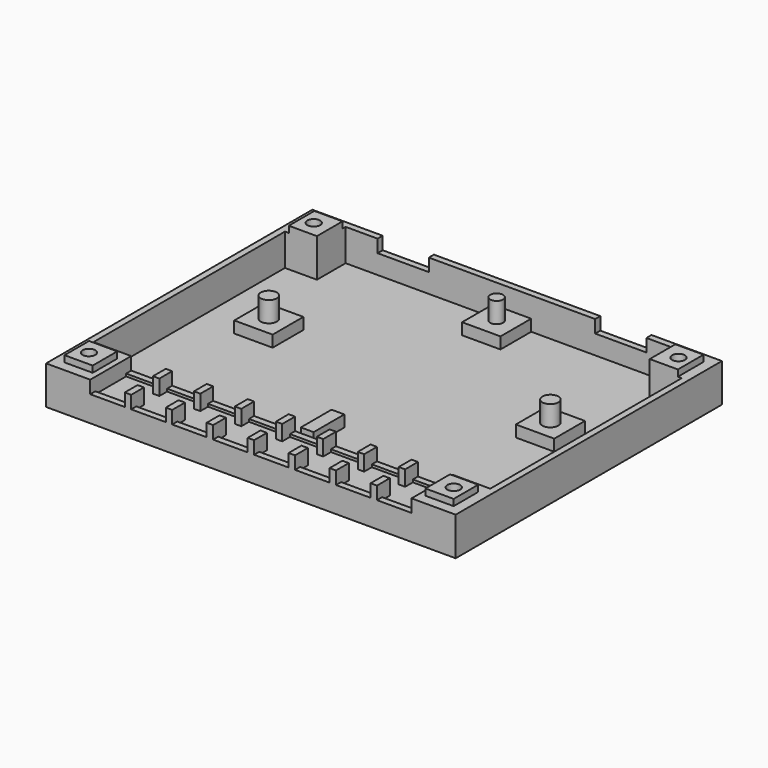
from build123d import *

# Parameters (mm, degrees)
F0_W          = 6.858
F0_H          = 3.81
F0_H_2        = 1.905
F0_W_2        = 1.27
F0_W_3        = 10.16
F0_H_3        = 13.335
F0_W_4        = 7.62
F0_H_4        = 7.62
F0_R          = 1.5875
F0_W_5        = 5.588
F0_H_5        = 6.096
F0_H_6        = 1.27
F0_R_2        = 1.27
F0_W_6        = 0.762
F0_H_7        = 6.35
F0_W_7        = 2.54
F1_DEPTH      = 5.08
F2_DEPTH      = 3.81
F3_DEPTH      = 1.524
F4_DEPTH      = 2.54
F5_DEPTH      = 2.54
F6_DEPTH      = 0.508
F7_DEPTH      = 3.81
F8_DEPTH      = 3.81
F8_DEPTH_BACK = 3.81


# Not quite as in the source:
# - a feature names something its author has since deleted; it is built from what else it names


with BuildPart() as f1:
    # F0 (on Top) → F1 (new body)
    with BuildSketch(Plane.XY):
        with Locations((4.064, -34.29)):
            Rectangle(F0_W, F0_H)
        with Locations((-20.32, -31.4325)):
            Rectangle(F0_W, F0_H_2)
        with Locations((28.448, -34.29)):
            Rectangle(F0_W, F0_H)
        with Locations((4.064, -37.1475)):
            Rectangle(F0_W, F0_H_2)
        with Locations((-4.064, -37.1475)):
            Rectangle(F0_W, F0_H_2)
        with Locations((0, -34.29)):
            Rectangle(F0_W_2, F0_H)
        with Locations((4.064, -31.4325)):
            Rectangle(F0_W, F0_H_2)
        with Locations((-4.064, -34.29)):
            Rectangle(F0_W, F0_H)
        with Locations((21.59, 18.7325)):
            Rectangle(F0_W_3, F0_H_3)
        with Locations((-21.59, 18.7325)):
            Rectangle(F0_W_3, F0_H_3)
        with Locations((-27.94, 0)):
            Rectangle(F0_W_4, F0_H_4)
        with Locations((-27.94, 0)):
            Circle(F0_R, mode=Mode.SUBTRACT)
        with Locations((27.94, 0)):
            Rectangle(F0_W_4, F0_H_4)
        with Locations((27.94, 0)):
            Circle(F0_R, mode=Mode.SUBTRACT)
        with Locations((-12.192, -37.1475)):
            Rectangle(F0_W, F0_H_2)
        Polygon((-3.81, 25.4), (-6.35, 25.4), (-16.51, 25.4), (-16.51, 12.065), (-26.67, 12.065), (-26.67, 25.4), (-31.75, 25.4), (-31.75, 3.81), (-24.13, 3.81), (-24.13, -3.81), (-31.75, -3.81), (-31.75, -25.4), (-1.27, -25.4), (-1.27, -17.78), (1.27, -17.78), (1.27, -25.4), (31.75, -25.4), (31.75, -3.81), (24.13, -3.81), (24.13, 3.81), (31.75, 3.81), (31.75, 25.4), (26.67, 25.4), (26.67, 12.065), (16.51, 12.065), (16.51, 25.4), (6.35, 25.4), (3.81, 25.4), (3.81, 17.78), (-3.81, 17.78), align=None)
        with Locations((-4.064, -31.4325)):
            Rectangle(F0_W, F0_H_2)
        with Locations((-16.256, -37.1475)):
            Rectangle(F0_W_2, F0_H_2)
        with Locations((-12.192, -34.29)):
            Rectangle(F0_W, F0_H)
        Polygon((40.64, 26.67), (26.67, 26.67), (26.67, 25.4), (31.75, 25.4), (33.02, 25.4), (39.37, 25.4), (39.37, 24.638), (39.37, 18.288), (39.37, -29.21), (31.877, -29.21), (31.877, -30.48), (39.37, -30.48), (39.37, -38.1), (31.877, -38.1), (31.877, -39.37), (40.64, -39.37), align=None)
        with Locations((-20.32, -37.1475)):
            Rectangle(F0_W, F0_H_2)
        with Locations((-20.32, -34.29)):
            Rectangle(F0_W, F0_H)
        Polygon((31.877, -36.195), (31.877, -38.1), (39.37, -38.1), (39.37, -30.48), (31.877, -30.48), (31.877, -32.385), align=None)
        with Locations((35.814, -34.29)):
            Rectangle(F0_W_5, F0_H_5, mode=Mode.SUBTRACT)
        with Locations((-12.192, -31.4325)):
            Rectangle(F0_W, F0_H_2)
        with Locations((12.192, -38.735)):
            Rectangle(F0_W, F0_H_6)
        with Locations((28.448, -38.735)):
            Rectangle(F0_W, F0_H_6)
        with Locations((28.448, -31.4325)):
            Rectangle(F0_W, F0_H_2)
        with Locations((-24.384, -34.29)):
            Rectangle(F0_W_2, F0_H)
        with Locations((20.32, -38.735)):
            Rectangle(F0_W, F0_H_6)
        with Locations((0, 21.59)):
            Rectangle(F0_W_4, F0_H_4)
        with Locations((0, 21.59)):
            Circle(F0_R_2, mode=Mode.SUBTRACT)
        with Locations((28.448, -37.1475)):
            Rectangle(F0_W, F0_H_2)
        with Locations((12.192, -37.1475)):
            Rectangle(F0_W, F0_H_2)
        with Locations((16.256, -34.29)):
            Rectangle(F0_W_2, F0_H)
        with Locations((-12.192, -38.735)):
            Rectangle(F0_W, F0_H_6)
        with Locations((-28.448, -31.4325)):
            Rectangle(F0_W, F0_H_2)
        with Locations((4.064, -38.735)):
            Rectangle(F0_W, F0_H_6)
        with Locations((20.32, -31.4325)):
            Rectangle(F0_W, F0_H_2)
        with Locations((20.32, -37.1475)):
            Rectangle(F0_W, F0_H_2)
        with Locations((12.192, -34.29)):
            Rectangle(F0_W, F0_H)
        with Locations((-20.32, -38.735)):
            Rectangle(F0_W, F0_H_6)
        with Locations((-28.448, -29.845)):
            Rectangle(F0_W, F0_H_6)
        with Locations((12.192, -31.4325)):
            Rectangle(F0_W, F0_H_2)
        with Locations((20.32, -34.29)):
            Rectangle(F0_W, F0_H)
        with Locations((-4.064, -38.735)):
            Rectangle(F0_W, F0_H_6)
        with Locations((12.192, -29.845)):
            Rectangle(F0_W, F0_H_6)
        with Locations((8.128, -34.29)):
            Rectangle(F0_W_2, F0_H)
        with Locations((0, -37.1475)):
            Rectangle(F0_W_2, F0_H_2)
        with Locations((24.384, -31.4325)):
            Rectangle(F0_W_2, F0_H_2)
        with Locations((4.064, -29.845)):
            Rectangle(F0_W, F0_H_6)
        with Locations((-38.989, 21.463)):
            Rectangle(F0_W_6, F0_H_7)
        with Locations((-35.814, 21.463)):
            Rectangle(F0_W_5, F0_H_7)
        with Locations((-36.195, 21.463)):
            Circle(F0_R_2, mode=Mode.SUBTRACT)
        with Locations((0, -21.59)):
            Rectangle(F0_W_7, F0_H_4)
        with Locations((38.989, 21.463)):
            Rectangle(F0_W_6, F0_H_7)
        with Locations((35.814, 21.463)):
            Rectangle(F0_W_5, F0_H_7)
        with Locations((36.195, 21.463)):
            Circle(F0_R_2, mode=Mode.SUBTRACT)
        with Locations((0, -31.4325)):
            Rectangle(F0_W_2, F0_H_2)
        with Locations((-8.128, -34.29)):
            Rectangle(F0_W_2, F0_H)
        with Locations((16.256, -37.1475)):
            Rectangle(F0_W_2, F0_H_2)
        with Locations((-4.064, -29.845)):
            Rectangle(F0_W, F0_H_6)
        with Locations((-16.256, -34.29)):
            Rectangle(F0_W_2, F0_H)
        with Locations((21.59, 26.035)):
            Rectangle(F0_W_3, F0_H_6)
        with Locations((-24.384, -37.1475)):
            Rectangle(F0_W_2, F0_H_2)
        with Locations((-21.59, 26.035)):
            Rectangle(F0_W_3, F0_H_6)
        with Locations((11.43, 26.035)):
            Rectangle(F0_W_3, F0_H_6)
        with Locations((-12.192, -29.845)):
            Rectangle(F0_W, F0_H_6)
        with Locations((-11.43, 26.035)):
            Rectangle(F0_W_3, F0_H_6)
        Polygon((-6.35, 26.67), (-6.35, 25.4), (-3.81, 25.4), (3.81, 25.4), (6.35, 25.4), (6.35, 26.67), align=None)
        with Locations((28.448, -29.845)):
            Rectangle(F0_W, F0_H_6)
        with Locations((16.256, -31.4325)):
            Rectangle(F0_W_2, F0_H_2)
        with Locations((24.384, -34.29)):
            Rectangle(F0_W_2, F0_H)
        with Locations((-20.32, -29.845)):
            Rectangle(F0_W, F0_H_6)
        with Locations((-24.384, -31.4325)):
            Rectangle(F0_W_2, F0_H_2)
        with Locations((20.32, -29.845)):
            Rectangle(F0_W, F0_H_6)
        with Locations((24.384, -37.1475)):
            Rectangle(F0_W_2, F0_H_2)
        with Locations((24.384, -29.845)):
            Rectangle(F0_W_2, F0_H_6)
        with Locations((24.384, -38.735)):
            Rectangle(F0_W_2, F0_H_6)
        with Locations((16.256, -29.845)):
            Rectangle(F0_W_2, F0_H_6)
        with Locations((16.256, -38.735)):
            Rectangle(F0_W_2, F0_H_6)
        with Locations((8.128, -29.845)):
            Rectangle(F0_W_2, F0_H_6)
        with Locations((-8.128, -37.1475)):
            Rectangle(F0_W_2, F0_H_2)
        with Locations((0, -29.845)):
            Rectangle(F0_W_2, F0_H_6)
        with Locations((8.128, -38.735)):
            Rectangle(F0_W_2, F0_H_6)
        with Locations((0, 21.59)):
            Circle(F0_R_2)
        with Locations((27.94, 0)):
            Circle(F0_R)
        with Locations((-27.94, 0)):
            Circle(F0_R)
        with Locations((0, -38.735)):
            Rectangle(F0_W_2, F0_H_6)
        with Locations((-8.128, -29.845)):
            Rectangle(F0_W_2, F0_H_6)
        with Locations((-16.256, -29.845)):
            Rectangle(F0_W_2, F0_H_6)
        with Locations((-8.128, -38.735)):
            Rectangle(F0_W_2, F0_H_6)
        with Locations((-16.256, -38.735)):
            Rectangle(F0_W_2, F0_H_6)
        with Locations((8.128, -31.4325)):
            Rectangle(F0_W_2, F0_H_2)
        with Locations((-8.128, -31.4325)):
            Rectangle(F0_W_2, F0_H_2)
        with Locations((-24.384, -38.735)):
            Rectangle(F0_W_2, F0_H_6)
        with Locations((-16.256, -31.4325)):
            Rectangle(F0_W_2, F0_H_2)
        with Locations((8.128, -37.1475)):
            Rectangle(F0_W_2, F0_H_2)
        with Locations((-24.384, -29.845)):
            Rectangle(F0_W_2, F0_H_6)
        with Locations((-28.448, -38.735)):
            Rectangle(F0_W, F0_H_6)
        Polygon((-31.75, 3.81), (-31.75, 25.4), (-33.02, 25.4), (-33.02, 24.638), (-33.02, 18.288), (-38.608, 18.288), (-39.37, 18.288), (-39.37, -29.21), (-31.877, -29.21), (-25.019, -29.21), (-23.749, -29.21), (-16.891, -29.21), (-15.621, -29.21), (-8.763, -29.21), (-7.493, -29.21), (-0.635, -29.21), (0.635, -29.21), (7.493, -29.21), (8.763, -29.21), (15.621, -29.21), (16.891, -29.21), (23.749, -29.21), (25.019, -29.21), (31.877, -29.21), (39.37, -29.21), (39.37, 18.288), (38.608, 18.288), (33.02, 18.288), (33.02, 24.638), (33.02, 25.4), (31.75, 25.4), (31.75, 3.81), (31.75, -3.81), (31.75, -25.4), (1.27, -25.4), (-1.27, -25.4), (-31.75, -25.4), (-31.75, -3.81), align=None)
        Polygon((-31.75, 25.4), (-26.67, 25.4), (-26.67, 26.67), (-40.64, 26.67), (-40.64, -39.37), (-31.877, -39.37), (-31.877, -38.1), (-39.37, -38.1), (-39.37, -30.48), (-31.877, -30.48), (-31.877, -29.21), (-39.37, -29.21), (-39.37, 18.288), (-39.37, 24.638), (-39.37, 25.4), (-33.02, 25.4), align=None)
        with Locations((-28.448, -37.1475)):
            Rectangle(F0_W, F0_H_2)
        with Locations((-28.448, -34.29)):
            Rectangle(F0_W, F0_H)
        Polygon((-39.37, -38.1), (-31.877, -38.1), (-31.877, -36.195), (-31.877, -32.385), (-31.877, -30.48), (-39.37, -30.48), align=None)
        with Locations((-35.814, -34.29)):
            Rectangle(F0_W_5, F0_H_5, mode=Mode.SUBTRACT)
        with Locations((-35.814, -34.29)):
            Rectangle(F0_W_5, F0_H_5)
        with Locations((-36.195, -34.29)):
            Circle(F0_R_2, mode=Mode.SUBTRACT)
        with Locations((35.814, -34.29)):
            Rectangle(F0_W_5, F0_H_5)
        with Locations((36.195, -34.29)):
            Circle(F0_R_2, mode=Mode.SUBTRACT)
        with Locations((-36.195, -34.29)):
            Circle(F0_R_2)
        with Locations((36.195, -34.29)):
            Circle(F0_R_2)
        Polygon((-33.02, 24.638), (-33.02, 25.4), (-39.37, 25.4), (-39.37, 24.638), (-38.608, 24.638), align=None)
        Polygon((39.37, 25.4), (33.02, 25.4), (33.02, 24.638), (38.608, 24.638), (39.37, 24.638), align=None)
        with Locations((-36.195, 21.463)):
            Circle(F0_R_2)
        with Locations((36.195, 21.463)):
            Circle(F0_R_2)
    extrude(amount=-F1_DEPTH)

    # F0 (on Top) → F2 (cut)
    with BuildSketch(Plane.XY):
        Polygon((-3.81, 25.4), (-6.35, 25.4), (-16.51, 25.4), (-16.51, 12.065), (-26.67, 12.065), (-26.67, 25.4), (-31.75, 25.4), (-31.75, 3.81), (-24.13, 3.81), (-24.13, -3.81), (-31.75, -3.81), (-31.75, -25.4), (-1.27, -25.4), (-1.27, -17.78), (1.27, -17.78), (1.27, -25.4), (31.75, -25.4), (31.75, -3.81), (24.13, -3.81), (24.13, 3.81), (31.75, 3.81), (31.75, 25.4), (26.67, 25.4), (26.67, 12.065), (16.51, 12.065), (16.51, 25.4), (6.35, 25.4), (3.81, 25.4), (3.81, 17.78), (-3.81, 17.78), align=None)
        with Locations((-21.59, 18.7325)):
            Rectangle(F0_W_3, F0_H_3)
        with Locations((21.59, 18.7325)):
            Rectangle(F0_W_3, F0_H_3)
        Polygon((-31.75, 3.81), (-31.75, 25.4), (-33.02, 25.4), (-33.02, 24.638), (-33.02, 18.288), (-38.608, 18.288), (-39.37, 18.288), (-39.37, -29.21), (-31.877, -29.21), (-25.019, -29.21), (-23.749, -29.21), (-16.891, -29.21), (-15.621, -29.21), (-8.763, -29.21), (-7.493, -29.21), (-0.635, -29.21), (0.635, -29.21), (7.493, -29.21), (8.763, -29.21), (15.621, -29.21), (16.891, -29.21), (23.749, -29.21), (25.019, -29.21), (31.877, -29.21), (39.37, -29.21), (39.37, 18.288), (38.608, 18.288), (33.02, 18.288), (33.02, 24.638), (33.02, 25.4), (31.75, 25.4), (31.75, 3.81), (31.75, -3.81), (31.75, -25.4), (1.27, -25.4), (-1.27, -25.4), (-31.75, -25.4), (-31.75, -3.81), align=None)
    extrude(amount=-F2_DEPTH, mode=Mode.SUBTRACT)

    # F0 (on Top) → F3 (cut)
    with BuildSketch(Plane.XY):
        with Locations((-27.94, 0)):
            Rectangle(F0_W_4, F0_H_4)
        with Locations((-27.94, 0)):
            Circle(F0_R, mode=Mode.SUBTRACT)
        with Locations((0, 21.59)):
            Rectangle(F0_W_4, F0_H_4)
        with Locations((0, 21.59)):
            Circle(F0_R_2, mode=Mode.SUBTRACT)
        with Locations((27.94, 0)):
            Rectangle(F0_W_4, F0_H_4)
        with Locations((27.94, 0)):
            Circle(F0_R, mode=Mode.SUBTRACT)
        with Locations((0, -21.59)):
            Rectangle(F0_W_7, F0_H_4)
    extrude(amount=-F3_DEPTH, mode=Mode.SUBTRACT)

    # F0 (on Top) → F4 (join)
    with BuildSketch(Plane.XY):
        with Locations((-27.94, 0)):
            Circle(F0_R)
        with Locations((27.94, 0)):
            Circle(F0_R)
        with Locations((0, 21.59)):
            Circle(F0_R_2)
        with Locations((-11.43, 26.035)):
            Rectangle(F0_W_3, F0_H_6)
        Polygon((-6.35, 26.67), (-6.35, 25.4), (-3.81, 25.4), (3.81, 25.4), (6.35, 25.4), (6.35, 26.67), align=None)
        with Locations((11.43, 26.035)):
            Rectangle(F0_W_3, F0_H_6)
    extrude(amount=F4_DEPTH)

    # F0 (on Top) → F5 (join)
    with BuildSketch(Plane.XY):
        Polygon((-31.75, 25.4), (-26.67, 25.4), (-26.67, 26.67), (-40.64, 26.67), (-40.64, -39.37), (-31.877, -39.37), (-31.877, -38.1), (-39.37, -38.1), (-39.37, -30.48), (-31.877, -30.48), (-31.877, -29.21), (-39.37, -29.21), (-39.37, 18.288), (-39.37, 24.638), (-39.37, 25.4), (-33.02, 25.4), align=None)
        with Locations((-24.384, -38.735)):
            Rectangle(F0_W_2, F0_H_6)
        with Locations((-24.384, -37.1475)):
            Rectangle(F0_W_2, F0_H_2)
        with Locations((-24.384, -31.4325)):
            Rectangle(F0_W_2, F0_H_2)
        with Locations((-24.384, -29.845)):
            Rectangle(F0_W_2, F0_H_6)
        with Locations((-16.256, -29.845)):
            Rectangle(F0_W_2, F0_H_6)
        with Locations((-8.128, -29.845)):
            Rectangle(F0_W_2, F0_H_6)
        with Locations((0, -29.845)):
            Rectangle(F0_W_2, F0_H_6)
        with Locations((8.128, -29.845)):
            Rectangle(F0_W_2, F0_H_6)
        with Locations((16.256, -29.845)):
            Rectangle(F0_W_2, F0_H_6)
        with Locations((16.256, -31.4325)):
            Rectangle(F0_W_2, F0_H_2)
        with Locations((8.128, -31.4325)):
            Rectangle(F0_W_2, F0_H_2)
        with Locations((0, -31.4325)):
            Rectangle(F0_W_2, F0_H_2)
        with Locations((-8.128, -31.4325)):
            Rectangle(F0_W_2, F0_H_2)
        with Locations((-16.256, -31.4325)):
            Rectangle(F0_W_2, F0_H_2)
        with Locations((-16.256, -37.1475)):
            Rectangle(F0_W_2, F0_H_2)
        with Locations((-8.128, -37.1475)):
            Rectangle(F0_W_2, F0_H_2)
        with Locations((0, -37.1475)):
            Rectangle(F0_W_2, F0_H_2)
        with Locations((8.128, -37.1475)):
            Rectangle(F0_W_2, F0_H_2)
        with Locations((16.256, -37.1475)):
            Rectangle(F0_W_2, F0_H_2)
        with Locations((8.128, -38.735)):
            Rectangle(F0_W_2, F0_H_6)
        with Locations((0, -38.735)):
            Rectangle(F0_W_2, F0_H_6)
        with Locations((-8.128, -38.735)):
            Rectangle(F0_W_2, F0_H_6)
        with Locations((-16.256, -38.735)):
            Rectangle(F0_W_2, F0_H_6)
        with Locations((16.256, -38.735)):
            Rectangle(F0_W_2, F0_H_6)
        with Locations((24.384, -38.735)):
            Rectangle(F0_W_2, F0_H_6)
        with Locations((24.384, -37.1475)):
            Rectangle(F0_W_2, F0_H_2)
        with Locations((24.384, -29.845)):
            Rectangle(F0_W_2, F0_H_6)
        with Locations((24.384, -31.4325)):
            Rectangle(F0_W_2, F0_H_2)
        Polygon((40.64, 26.67), (26.67, 26.67), (26.67, 25.4), (31.75, 25.4), (33.02, 25.4), (39.37, 25.4), (39.37, 24.638), (39.37, 18.288), (39.37, -29.21), (31.877, -29.21), (31.877, -30.48), (39.37, -30.48), (39.37, -38.1), (31.877, -38.1), (31.877, -39.37), (40.64, -39.37), align=None)
        Polygon((-39.37, -38.1), (-31.877, -38.1), (-31.877, -36.195), (-31.877, -32.385), (-31.877, -30.48), (-39.37, -30.48), align=None)
        with Locations((-35.814, -34.29)):
            Rectangle(F0_W_5, F0_H_5, mode=Mode.SUBTRACT)
        Polygon((31.877, -36.195), (31.877, -38.1), (39.37, -38.1), (39.37, -30.48), (31.877, -30.48), (31.877, -32.385), align=None)
        with Locations((35.814, -34.29)):
            Rectangle(F0_W_5, F0_H_5, mode=Mode.SUBTRACT)
        with Locations((-38.989, 21.463)):
            Rectangle(F0_W_6, F0_H_7)
        Polygon((-33.02, 24.638), (-33.02, 25.4), (-39.37, 25.4), (-39.37, 24.638), (-38.608, 24.638), align=None)
        Polygon((39.37, 25.4), (33.02, 25.4), (33.02, 24.638), (38.608, 24.638), (39.37, 24.638), align=None)
        with Locations((38.989, 21.463)):
            Rectangle(F0_W_6, F0_H_7)
    extrude(amount=F5_DEPTH)

    # F0 (on Top) → F6 (cut)
    with BuildSketch(Plane.XY):
        with Locations((-28.448, -31.4325)):
            Rectangle(F0_W, F0_H_2)
        with Locations((-28.448, -34.29)):
            Rectangle(F0_W, F0_H)
        with Locations((-28.448, -37.1475)):
            Rectangle(F0_W, F0_H_2)
        with Locations((-24.384, -34.29)):
            Rectangle(F0_W_2, F0_H)
        with Locations((-20.32, -31.4325)):
            Rectangle(F0_W, F0_H_2)
        with Locations((-20.32, -34.29)):
            Rectangle(F0_W, F0_H)
        with Locations((-20.32, -37.1475)):
            Rectangle(F0_W, F0_H_2)
        with Locations((-16.256, -34.29)):
            Rectangle(F0_W_2, F0_H)
        with Locations((-12.192, -34.29)):
            Rectangle(F0_W, F0_H)
        with Locations((-12.192, -31.4325)):
            Rectangle(F0_W, F0_H_2)
        with Locations((-12.192, -37.1475)):
            Rectangle(F0_W, F0_H_2)
        with Locations((-4.064, -31.4325)):
            Rectangle(F0_W, F0_H_2)
        with Locations((-8.128, -34.29)):
            Rectangle(F0_W_2, F0_H)
        with Locations((-4.064, -34.29)):
            Rectangle(F0_W, F0_H)
        with Locations((-4.064, -37.1475)):
            Rectangle(F0_W, F0_H_2)
        with Locations((4.064, -31.4325)):
            Rectangle(F0_W, F0_H_2)
        with Locations((4.064, -34.29)):
            Rectangle(F0_W, F0_H)
        with Locations((0, -34.29)):
            Rectangle(F0_W_2, F0_H)
        with Locations((4.064, -37.1475)):
            Rectangle(F0_W, F0_H_2)
        with Locations((8.128, -34.29)):
            Rectangle(F0_W_2, F0_H)
        with Locations((12.192, -31.4325)):
            Rectangle(F0_W, F0_H_2)
        with Locations((12.192, -34.29)):
            Rectangle(F0_W, F0_H)
        with Locations((12.192, -37.1475)):
            Rectangle(F0_W, F0_H_2)
        with Locations((20.32, -31.4325)):
            Rectangle(F0_W, F0_H_2)
        with Locations((16.256, -34.29)):
            Rectangle(F0_W_2, F0_H)
        with Locations((20.32, -34.29)):
            Rectangle(F0_W, F0_H)
        with Locations((20.32, -37.1475)):
            Rectangle(F0_W, F0_H_2)
        with Locations((28.448, -31.4325)):
            Rectangle(F0_W, F0_H_2)
        with Locations((24.384, -34.29)):
            Rectangle(F0_W_2, F0_H)
        with Locations((28.448, -34.29)):
            Rectangle(F0_W, F0_H)
        with Locations((28.448, -37.1475)):
            Rectangle(F0_W, F0_H_2)
    extrude(amount=-F6_DEPTH, mode=Mode.SUBTRACT)

    # F0 (on Top) → F7 (join)
    with BuildSketch(Plane.XY):
        with Locations((-35.814, 21.463)):
            Rectangle(F0_W_5, F0_H_7)
        with Locations((-36.195, 21.463)):
            Circle(F0_R_2, mode=Mode.SUBTRACT)
        with Locations((35.814, 21.463)):
            Rectangle(F0_W_5, F0_H_7)
        with Locations((36.195, 21.463)):
            Circle(F0_R_2, mode=Mode.SUBTRACT)
        with Locations((35.814, -34.29)):
            Rectangle(F0_W_5, F0_H_5)
        with Locations((36.195, -34.29)):
            Circle(F0_R_2, mode=Mode.SUBTRACT)
        with Locations((-35.814, -34.29)):
            Rectangle(F0_W_5, F0_H_5)
        with Locations((-36.195, -34.29)):
            Circle(F0_R_2, mode=Mode.SUBTRACT)
        with Locations((-36.195, -34.29)):
            Circle(F0_R_2)
        with Locations((36.195, -34.29)):
            Circle(F0_R_2)
        with Locations((-36.195, 21.463)):
            Circle(F0_R_2)
        with Locations((36.195, 21.463)):
            Circle(F0_R_2)
    extrude(amount=F7_DEPTH)

    # F0 (on Top) → F8 (cut, two sides)
    with BuildSketch(Plane.XY) as f8_sk:
        with Locations((-36.195, 21.463)):
            Circle(F0_R_2)
        with Locations((36.195, 21.463)):
            Circle(F0_R_2)
        with Locations((36.195, -34.29)):
            Circle(F0_R_2)
        with Locations((-36.195, -34.29)):
            Circle(F0_R_2)
    extrude(amount=F8_DEPTH, mode=Mode.SUBTRACT)
    extrude(f8_sk.sketch, amount=-F8_DEPTH_BACK, mode=Mode.SUBTRACT)


solid = f1.part
